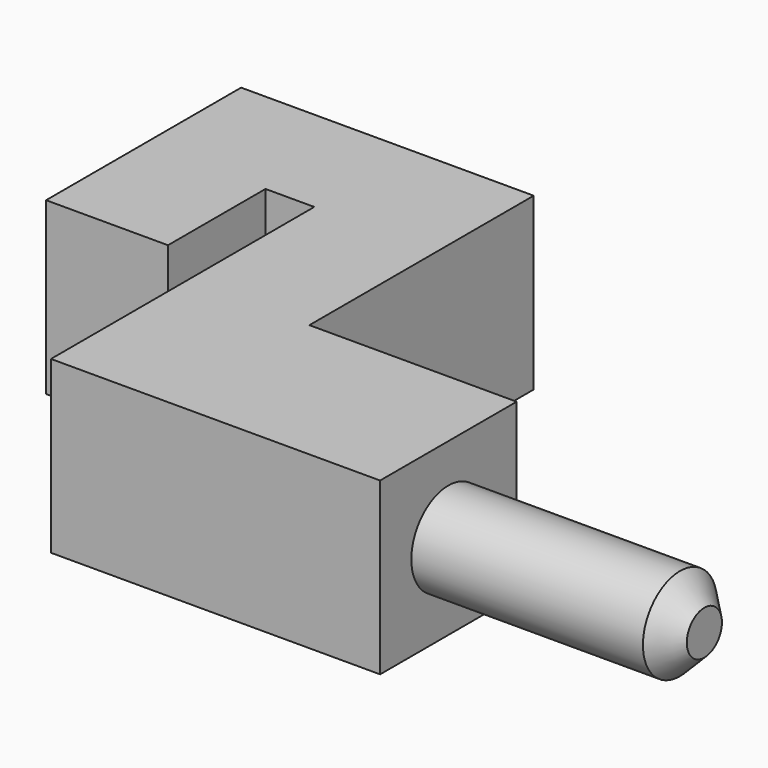
from build123d import *

# Parameters (mm, degrees)
F1_DEPTH = 7
F2_R     = 1.9
F3_DEPTH = 10.5
F4_SIZE  = 1


# Not quite as in the source:
# - a feature names something its author has since deleted; it is built from what else it names


with BuildPart() as f1:
    # F0 (on Top) → F1 (new body)
    with BuildSketch(Plane.XY):
        Polygon((0, 18.5), (0, 8.5), (5, 8.5), (5, 13.5), (7, 13.5), (7, 0), (20.5, 0), (20.5, 7), (12, 7), (12, 18.5), align=None)
    extrude(amount=F1_DEPTH)

    # F2 (on face) → F3 (join)
    with BuildSketch(Plane.YZ.offset(20.5)):
        with Locations((3.5, 3.5)):
            Circle(F2_R)
    extrude(amount=F3_DEPTH)

    # F4
    f4_edges = [f1.edges().sort_by_distance(p)[0] for p in [
        (31, 1.6, 3.5),
    ]]
    chamfer(f4_edges, length=F4_SIZE)


solid = f1.part
